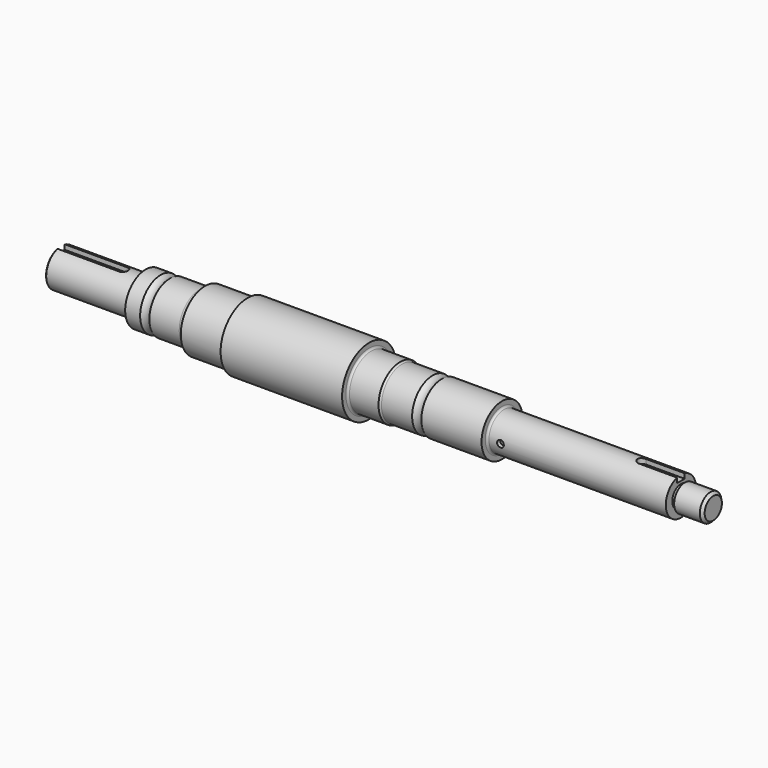
from build123d import *

# Parameters (mm, degrees)
F2_SIZE   = 0.5
F3_R      = 2
F5_R      = 1.5
F6_R      = 1.5
F8_SIZE   = 2
F11_DEPTH = 4
F13_DEPTH = 4
F16_DEPTH = 3
F19_DEPTH = 3


# Not quite as in the source:
# - a fillet or chamfer that OpenCascade refuses, or shapes differently, is made with other operations: its cross-section is extruded or revolved along the edge and cut away or added


with BuildPart() as f1:
    # F0 (on Front) → F1 (revolve)
    with BuildSketch(Plane.XZ):
        with BuildLine():
            Line((63, 14), (0, 14))
            Line((0, 14), (0, 0))
            Line((0, 0), (483.5, 0))
            Line((483.5, 0), (483.5, 10))
            Line((483.5, 10), (462.5, 10))
            Line((462.5, 10), (462.5, 8))
            Line((462.5, 8), (459.5, 8))
            Line((459.5, 8), (459.5, 14))
            Line((459.5, 14), (327, 14))
            Line((327, 14), (327, 19))
            Line((327, 19), (282.4058772732, 19))
            ThreePointArc((282.4058772732, 19), (279, 18), (275.5941227268, 19))
            Line((275.5941227268, 19), (251.5, 19))
            Line((251.5, 19), (251.5, 20))
            Line((251.5, 20), (228.5, 20))
            Line((228.5, 20), (228.5, 25))
            Line((228.5, 25), (138.5, 25))
            Line((138.5, 25), (138.5, 22.5))
            Line((138.5, 22.5), (107, 22.5))
            Line((107, 22.5), (107, 19))
            Line((107, 19), (80.9058772732, 19))
            ThreePointArc((80.9058772732, 19), (77.5, 18), (74.0941227268, 19))
            Line((74.0941227268, 19), (63, 19))
            Line((63, 19), (63, 14))
        make_face()
    revolve(axis=Axis((247.1050164511, 0, 0), (1, 0, 0)))

    # F2
    f2_edges = [f1.edges().sort_by_distance(p)[0] for p in [
        (0, 0, -14),
    ]]
    chamfer(f2_edges, length=F2_SIZE)

    # F3
    f3_edges = [f1.edges().sort_by_distance(p)[0] for p in [
        (63, 0, -14),
    ]]
    fillet(f3_edges, radius=F3_R)

    # F4: fillet of radius 4 on 1 edges, made by hand

    # F4_s1 → F4_t2 (revolve)
    with BuildSketch(Plane.XZ):
        with BuildLine():
            ThreePointArc((103.0313730334, 19), (105.6771243445, 20), (107, 22.5))
            Line((107, 22.5), (107, 19))
            Line((107, 19), (103.0313730334, 19))
        make_face()
    revolve(axis=Axis((107, 0, 0), (1, 0, 0)))

    # F5
    f5_edges = [f1.edges().sort_by_distance(p)[0] for p in [
        (138.5, 0, -22.5),
    ]]
    fillet(f5_edges, radius=F5_R)

    # F6
    f6_edges = [f1.edges().sort_by_distance(p)[0] for p in [
        (228.5, 0, -20),
    ]]
    fillet(f6_edges, radius=F6_R)

    # F7: fillet of radius 1.5 on 2 edges, made by hand

    # F7_s1 → F7_t2 (revolve)
    with BuildSketch(Plane.XZ):
        with BuildLine():
            ThreePointArc((251.5, 20), (252.0481881586, 19.2752551286), (252.9142135624, 19))
            Line((252.9142135624, 19), (251.5, 19))
            Line((251.5, 19), (251.5, 20))
        make_face()
    revolve(axis=Axis((251.5, 0, 0), (1, 0, 0)))

    # F7_s3 → F7_t4 (revolve)
    with BuildSketch(Plane.XZ):
        with BuildLine():
            ThreePointArc((327, 15.5), (327.4393398282, 14.4393398282), (328.5, 14))
            Line((328.5, 14), (327, 14))
            Line((327, 14), (327, 15.5))
        make_face()
    revolve(axis=Axis((327, 0, 0), (1, 0, 0)))

    # F8
    f8_edges = [f1.edges().sort_by_distance(p)[0] for p in [
        (483.5, 0, -10),
    ]]
    chamfer(f8_edges, length=F8_SIZE)

    # F10 (on offset) → F11 (cut)
    with BuildSketch(Plane.XY.offset(14)):
        with BuildLine():
            Line((46.5, 3.5), (0, 3.5))
            Line((0, 3.5), (0, -3.5))
            Line((0, -3.5), (46.5, -3.5))
            ThreePointArc((46.5, -3.5), (50, 0), (46.5, 3.5))
        make_face()
    extrude(amount=-F11_DEPTH, mode=Mode.SUBTRACT)

    # F12 (on offset) → F13 (cut)
    with BuildSketch(Plane.XY.offset(14)):
        with BuildLine():
            Line((431, -3.5), (459.5, -3.5))
            Line((459.5, -3.5), (459.5, 3.5))
            Line((459.5, 3.5), (431, 3.5))
            ThreePointArc((431, 3.5), (427.5, 0), (431, -3.5))
        make_face()
    extrude(amount=-F13_DEPTH, mode=Mode.SUBTRACT)

    # F15 (on offset) → F16 (cut)
    with BuildSketch(Plane.XZ.offset(14)):
        with BuildLine():
            ThreePointArc((334.5, 0), (337, -2.5), (339.5, 0))
            Line((339.5, 0), (334.5, 0))
        make_face()
        with BuildLine():
            Line((334.5, 0), (339.5, 0))
            ThreePointArc((339.5, 0), (337, 2.5), (334.5, 0))
        make_face()
    extrude(amount=-F16_DEPTH, mode=Mode.SUBTRACT)

    # F18 (on offset) → F19 (cut)
    with BuildSketch(Plane.XY.offset(-14)):
        with BuildLine():
            ThreePointArc((339.5, 0), (337, 2.5), (334.5, 0))
            Line((334.5, 0), (339.5, 0))
        make_face()
        with BuildLine():
            Line((339.5, 0), (334.5, 0))
            ThreePointArc((334.5, 0), (337, -2.5), (339.5, 0))
        make_face()
    extrude(amount=F19_DEPTH, mode=Mode.SUBTRACT)


solid = f1.part
